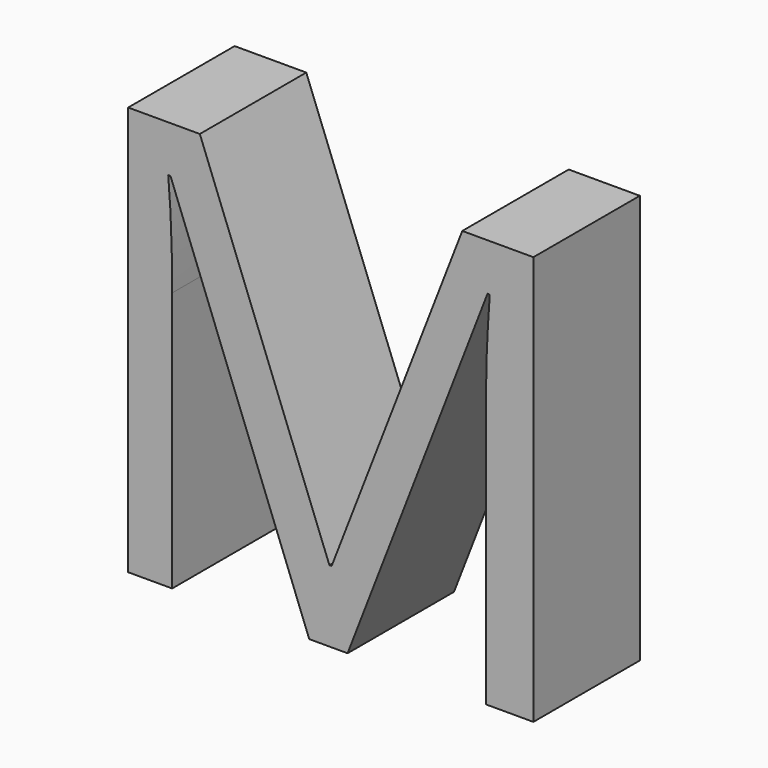
from build123d import *

# Parameters (mm, degrees)
F0_TEXT_SIZE = 43.0734188538
F1_DEPTH     = 10


# Not quite as in the source:
# - Text() gives the source's letters only with a copy of the font that has no kerning and outlines rounded to 1/6400 em; it was checked with that copy


with BuildPart() as f1:
    # F0 (on Front) → F1 (new body)
    with BuildSketch(Plane.XZ):
        with Locations((-37.4738744028, 0)):
            Text('M', F0_TEXT_SIZE, font='Open Sans', text_align=(TextAlign.LEFT, TextAlign.BOTTOM))
    extrude(amount=F1_DEPTH)


solid = f1.part
